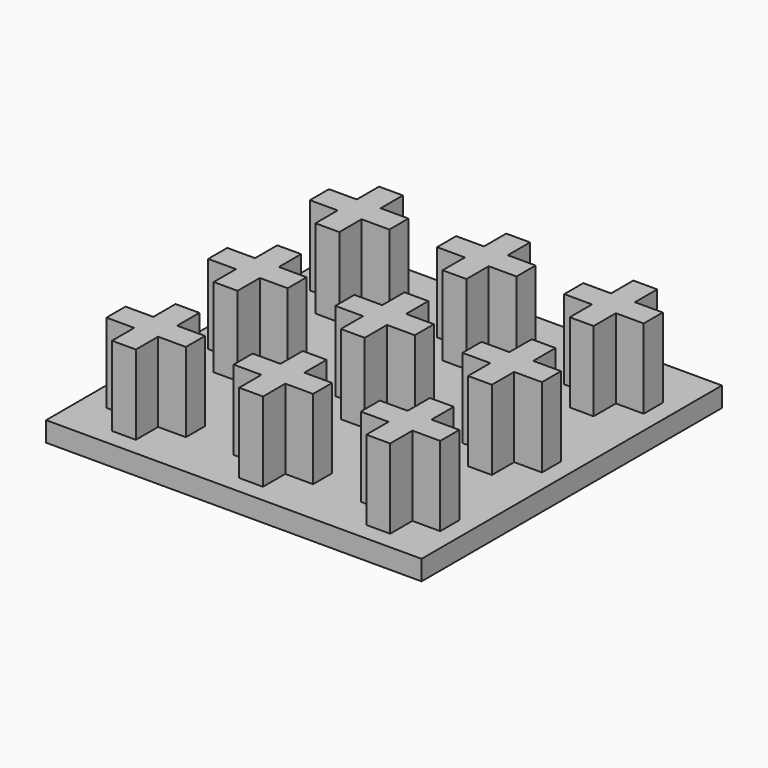
from build123d import *

# Parameters (mm, degrees)
F0_W         = 120
F0_H         = 120
F1_DEPTH     = 6.35
F2_W         = 7.62
F2_H         = 8.89
F2_H_2       = 7.62
F2_W_2       = 8.89
F3_DEPTH     = 25.4
F4_TEXT_SIZE = 5.2048937909
F5_DEPTH     = 3.81


# Not quite as in the source:
# - Text() gives the source's letters only with a copy of the font that has no kerning and outlines rounded to 1/6400 em; it was checked with that copy


with BuildPart() as f1:
    # F0 (on Top) → F1 (new body)
    with BuildSketch(Plane.XY):
        with Locations((2.342062071, 11.9029206019)):
            Rectangle(F0_W, F0_H)
    extrude(amount=F1_DEPTH)

    # F2 (on face) → F3 (join)
    with BuildSketch(Plane.XY.offset(6.35)):
        with Locations((-37.337937929, 59.8379206019)):
            Rectangle(F2_W, F2_H)
        with Locations((-37.337937929, 51.5829206019)):
            Rectangle(F2_W, F2_H_2)
        with Locations((-45.592937929, 51.5829206019)):
            Rectangle(F2_W_2, F2_H_2)
        with Locations((-29.082937929, 51.5829206019)):
            Rectangle(F2_W_2, F2_H_2)
        with Locations((-37.337937929, 43.3279206019)):
            Rectangle(F2_W, F2_H)
        with Locations((-29.082937929, 10.9429206019)):
            Rectangle(F2_W_2, F2_H_2)
        with Locations((-37.337937929, 19.1979206019)):
            Rectangle(F2_W, F2_H)
        with Locations((-37.337937929, 10.9429206019)):
            Rectangle(F2_W, F2_H_2)
        with Locations((-37.337937929, 2.6879206019)):
            Rectangle(F2_W, F2_H)
        with Locations((-45.592937929, 10.9429206019)):
            Rectangle(F2_W_2, F2_H_2)
        with Locations((-29.082937929, -29.6970793981)):
            Rectangle(F2_W_2, F2_H_2)
        with Locations((-37.337937929, -21.4420793981)):
            Rectangle(F2_W, F2_H)
        with Locations((-37.337937929, -29.6970793981)):
            Rectangle(F2_W, F2_H_2)
        with Locations((-37.337937929, -37.9520793981)):
            Rectangle(F2_W, F2_H)
        with Locations((-45.592937929, -29.6970793981)):
            Rectangle(F2_W_2, F2_H_2)
        with Locations((11.557062071, 51.5829206019)):
            Rectangle(F2_W_2, F2_H_2)
        with Locations((3.302062071, 59.8379206019)):
            Rectangle(F2_W, F2_H)
        with Locations((3.302062071, 51.5829206019)):
            Rectangle(F2_W, F2_H_2)
        with Locations((3.302062071, 43.3279206019)):
            Rectangle(F2_W, F2_H)
        with Locations((-4.952937929, 51.5829206019)):
            Rectangle(F2_W_2, F2_H_2)
        with Locations((11.557062071, 10.9429206019)):
            Rectangle(F2_W_2, F2_H_2)
        with Locations((3.302062071, 19.1979206019)):
            Rectangle(F2_W, F2_H)
        with Locations((3.302062071, 10.9429206019)):
            Rectangle(F2_W, F2_H_2)
        with Locations((3.302062071, 2.6879206019)):
            Rectangle(F2_W, F2_H)
        with Locations((-4.952937929, 10.9429206019)):
            Rectangle(F2_W_2, F2_H_2)
        with Locations((11.557062071, -29.6970793981)):
            Rectangle(F2_W_2, F2_H_2)
        with Locations((3.302062071, -21.4420793981)):
            Rectangle(F2_W, F2_H)
        with Locations((3.302062071, -29.6970793981)):
            Rectangle(F2_W, F2_H_2)
        with Locations((3.302062071, -37.9520793981)):
            Rectangle(F2_W, F2_H)
        with Locations((-4.952937929, -29.6970793981)):
            Rectangle(F2_W_2, F2_H_2)
        with Locations((52.197062071, 51.5829206019)):
            Rectangle(F2_W_2, F2_H_2)
        with Locations((43.942062071, 59.8379206019)):
            Rectangle(F2_W, F2_H)
        with Locations((43.942062071, 51.5829206019)):
            Rectangle(F2_W, F2_H_2)
        with Locations((43.942062071, 43.3279206019)):
            Rectangle(F2_W, F2_H)
        with Locations((35.687062071, 51.5829206019)):
            Rectangle(F2_W_2, F2_H_2)
        with Locations((52.197062071, 10.9429206019)):
            Rectangle(F2_W_2, F2_H_2)
        with Locations((43.942062071, 19.1979206019)):
            Rectangle(F2_W, F2_H)
        with Locations((43.942062071, 10.9429206019)):
            Rectangle(F2_W, F2_H_2)
        with Locations((43.942062071, 2.6879206019)):
            Rectangle(F2_W, F2_H)
        with Locations((35.687062071, 10.9429206019)):
            Rectangle(F2_W_2, F2_H_2)
        with Locations((52.197062071, -29.6970793981)):
            Rectangle(F2_W_2, F2_H_2)
        with Locations((43.942062071, -21.4420793981)):
            Rectangle(F2_W, F2_H)
        with Locations((43.942062071, -29.6970793981)):
            Rectangle(F2_W, F2_H_2)
        with Locations((43.942062071, -37.9520793981)):
            Rectangle(F2_W, F2_H)
        with Locations((35.687062071, -29.6970793981)):
            Rectangle(F2_W_2, F2_H_2)
    extrude(amount=F3_DEPTH)

    # F4 (on face) → F5 (join)
    with BuildSketch(Plane.XY.offset(6.35)):
        Polygon((-18.0812195957, -6.1508544228), (-21.2562195957, -6.1508544228), (-21.2562195957, -14.6334366873), (-12.9904156609, -14.6334366873), (-12.9904156609, -11.4584366873), (-18.0812195957, -11.4584366873), align=None)
        Polygon((-23.1612195957, -6.1508544228), (-21.2562195957, -6.1508544228), (-18.0812195957, -6.1508544228), (-16.1762195957, -6.1508544228), (-19.6687195957, -2.9758544228), align=None)
        Polygon((-12.9904156609, -11.4584366873), (-12.9904156609, -14.6334366873), (-12.9904156609, -16.5384366873), (-9.8154156609, -13.0459366873), (-12.9904156609, -9.5534366873), align=None)
        with Locations((-21.0745056856, -0.5260034054)):
            Text('Y', F4_TEXT_SIZE, font='Open Sans', text_align=(TextAlign.LEFT, TextAlign.BOTTOM))
        with Locations((-7.8082897189, -15.2039140052)):
            Text('X', F4_TEXT_SIZE, font='Open Sans', text_align=(TextAlign.LEFT, TextAlign.BOTTOM))
    extrude(amount=F5_DEPTH)


solid = f1.part
